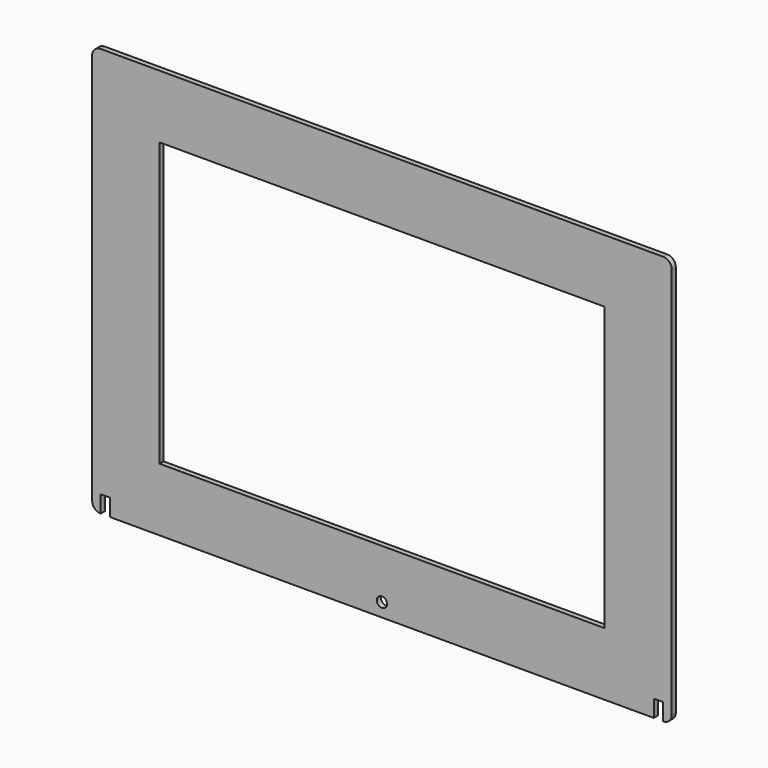
from build123d import *

# Parameters (mm, degrees)
F1_DEPTH = 3
F2_W     = 261
F2_H     = 166
F2_R     = 3
F3_DEPTH = 3
F4_R     = 4.99999


# Not quite as in the source:
# - a fillet or chamfer is up to 0.001 mm smaller than in the source, because OpenCascade refuses the exact size


with BuildPart() as f1:
    # F0 (on Front) → F1 (new body)
    with BuildSketch(Plane.XZ):
        Polygon((170, -120), (170, 120), (-170, 120), (-170, -120), (-165, -120), (-165, -110), (-159.5, -110), (-159.5, -120), (159.5, -120), (159.5, -110), (165, -110), (165, -120), align=None)
    extrude(amount=F1_DEPTH)

    # F2 (on face) → F3 (cut, through all)
    with BuildSketch(Plane.XZ.offset(3)):
        Rectangle(F2_W, F2_H)
        with Locations((0, -112)):
            Circle(F2_R)
    extrude(amount=-F3_DEPTH, mode=Mode.SUBTRACT)

    # F4 (radius 5 in the source; OpenCascade refuses exactly that, so slightly less here)
    f4_edges = [f1.edges().sort_by_distance(p)[0] for p in [
        (-170, -1.5, 120),
        (170, -1.5, 120),
        (170, -1.5, -120),
        (-170, -1.5, -120),
    ]]
    fillet(f4_edges, radius=F4_R)


solid = f1.part
